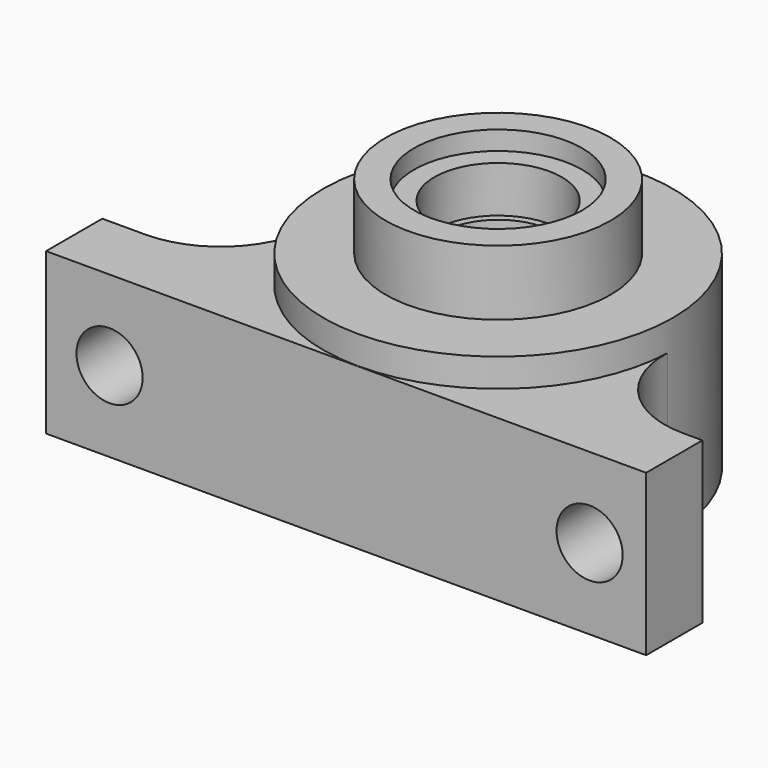
from build123d import *

# Parameters (mm, degrees)
F1_DEPTH    = 17
F3_DEPTH    = 9.5
F4_DEPTH    = 2
F5_R        = 15.5
F5_R_2      = 6
F6_DEPTH    = 3
F7_R        = 11.9
F7_R_2      = 8.9
F8_DEPTH    = 6.9
F9_T1_DEPTH = 17
F10_R       = 3.5
F11_DEPTH   = 37.0302756021
F13_DEPTH   = 29.5909779782
F14_R       = 6
F15_DEPTH   = 29.5909779782
F7_R_3      = 6.75
F16_DEPTH   = 4.9


# Not quite as in the source:
# - a fillet or chamfer that OpenCascade refuses, or shapes differently, is made with other operations: its cross-section is extruded or revolved along the edge and cut away or added
# - a feature names something its author has since deleted; it is built from what else it names


with BuildPart() as f1:
    # F0 (on Top) → F1 (new body)
    with BuildSketch(Plane.XY):
        with BuildLine():
            ThreePointArc((0, -15.5), (-5.8461671777, -14.3552195849), (-10.8287759439, -11.0899779782))
            Line((-10.8287759439, -11.0899779782), (-14.8075112171, -11.0899779782))
            ThreePointArc((-14.8075112171, -11.0899779782), (-12.6472106411, -13.5017799938), (-10.0995049384, -15.5))
            Line((-10.0995049384, -15.5), (0, -15.5))
        make_face()
        with BuildLine():
            Line((14.8075112171, -11.0899779782), (10.8287759439, -11.0899779782))
            ThreePointArc((10.8287759439, -11.0899779782), (5.8461671777, -14.3552195849), (0, -15.5))
            Line((0, -15.5), (10.0995049384, -15.5))
            ThreePointArc((10.0995049384, -15.5), (12.6472106411, -13.5017799938), (14.8075112171, -11.0899779782))
        make_face()
        with BuildLine():
            ThreePointArc((-10.8287759439, -11.0899779782), (-6.0168086586, 14.2845375692), (15.5, 0))
            ThreePointArc((15.5, 0), (14.2845375692, -6.0168086586), (10.8287759439, -11.0899779782))
            Line((10.8287759439, -11.0899779782), (14.8075112171, -11.0899779782))
            ThreePointArc((14.8075112171, -11.0899779782), (17.5526202818, -5.8442725161), (18.5, 0))
            ThreePointArc((18.5, 0), (-5.8442725161, 17.5526202818), (-14.8075112171, -11.0899779782))
            Line((-14.8075112171, -11.0899779782), (-10.8287759439, -11.0899779782))
        make_face()
        with BuildLine():
            Line((30.4899009168, -15.5), (10.0995049384, -15.5))
            ThreePointArc((10.0995049384, -15.5), (0, -18.5), (-10.0995049384, -15.5))
            Line((-10.0995049384, -15.5), (-33.0100990832, -15.5))
            Line((-33.0100990832, -15.5), (-33.0100990832, -18.5292756021))
            Line((-33.0100990832, -18.5292756021), (30.4899009168, -18.5292756021))
            Line((30.4899009168, -18.5292756021), (30.4899009168, -15.5))
        make_face()
        with BuildLine():
            Line((30.4899009168, -11.0899779782), (14.8075112171, -11.0899779782))
            ThreePointArc((14.8075112171, -11.0899779782), (12.6472106411, -13.5017799938), (10.0995049384, -15.5))
            Line((10.0995049384, -15.5), (30.4899009168, -15.5))
            Line((30.4899009168, -15.5), (30.4899009168, -11.0899779782))
        make_face()
        with BuildLine():
            ThreePointArc((-10.0995049384, -15.5), (-12.6472106411, -13.5017799938), (-14.8075112171, -11.0899779782))
            Line((-14.8075112171, -11.0899779782), (-33.0100990832, -11.0899779782))
            Line((-33.0100990832, -11.0899779782), (-33.0100990832, -15.5))
            Line((-33.0100990832, -15.5), (-10.0995049384, -15.5))
        make_face()
        with BuildLine():
            Line((10.0995049384, -15.5), (0, -15.5))
            Line((0, -15.5), (-10.0995049384, -15.5))
            ThreePointArc((-10.0995049384, -15.5), (0, -18.5), (10.0995049384, -15.5))
        make_face()
    extrude(amount=F1_DEPTH)

    # F5 (on face) → F6 (join)
    with BuildSketch(Plane.XY.offset(17)):
        with BuildLine():
            ThreePointArc((14.8075112171, -11.0899779782), (17.5526202818, -5.8442725161), (18.5, 0))
            ThreePointArc((18.5, 0), (-5.8442725161, 17.5526202818), (-14.8075112171, -11.0899779782))
            ThreePointArc((-14.8075112171, -11.0899779782), (0, -18.5), (14.8075112171, -11.0899779782))
        make_face()
        Circle(F5_R, mode=Mode.SUBTRACT)
        Circle(F5_R)
        Circle(F5_R_2, mode=Mode.SUBTRACT)
    extrude(amount=F6_DEPTH)

    # F7 (on face) → F8 (join)
    with BuildSketch(Plane.XY.offset(20)):
        Circle(F7_R)
        Circle(F7_R_2, mode=Mode.SUBTRACT)
    extrude(amount=F8_DEPTH)

    # F9: fillet of radius 10 on 2 edges, made by hand

    # F9_s2 → F9_t1 (join)
    with BuildSketch(Plane.XY):
        with BuildLine():
            ThreePointArc((18.486465371, -0.7075295648), (21.2741342918, -8.0245116996), (28.4791493554, -11.0899779782))
            Line((28.4791493554, -11.0899779782), (14.8075112171, -11.0899779782))
            ThreePointArc((14.8075112171, -11.0899779782), (17.4376325236, -6.1789134946), (18.486465371, -0.7075295648))
        make_face()
        with BuildLine():
            ThreePointArc((-18.486465371, -0.7075295648), (-21.2741342918, -8.0245116996), (-28.4791493554, -11.0899779782))
            Line((-28.4791493554, -11.0899779782), (-14.8075112171, -11.0899779782))
            ThreePointArc((-14.8075112171, -11.0899779782), (-17.4376325236, -6.1789134946), (-18.486465371, -0.7075295648))
        make_face()
    extrude(amount=F9_T1_DEPTH)

    # F10 (on face) → F11 (cut, through all)
    with BuildSketch(Plane.XZ.offset(18.5292756021)):
        with Locations((-26.2949950993, 8.5148541257)):
            Circle(F10_R)
        with Locations((24.5050049007, 8.5148541257)):
            Circle(F10_R)
    extrude(amount=-F11_DEPTH, mode=Mode.SUBTRACT)

    # F12 (on face) → F13 (cut, through all)
    with BuildSketch(Plane(origin=(0, -11.0899779782, 0), x_dir=(-1, 0, 0), z_dir=(0, 1, 0))):
        with BuildLine():
            Line((28.4791493554, 11.2497161305), (28.4791493554, 14.1031875253))
            ThreePointArc((28.4791493554, 14.1031875253), (20.2949950993, 8.5148541257), (28.4791493554, 2.926520726))
            Line((28.4791493554, 2.926520726), (28.4791493554, 5.7799921208))
            ThreePointArc((28.4791493554, 5.7799921208), (29.7949950993, 8.5148541257), (28.4791493554, 11.2497161305))
        make_face()
        with BuildLine():
            ThreePointArc((28.4791493554, 2.926520726), (31.2500392735, 5.1314331894), (32.2949950993, 8.5148541257))
            ThreePointArc((32.2949950993, 8.5148541257), (31.2500392735, 11.8982750619), (28.4791493554, 14.1031875253))
            Line((28.4791493554, 14.1031875253), (28.4791493554, 11.2497161305))
            ThreePointArc((28.4791493554, 11.2497161305), (29.7949950993, 8.5148541257), (28.4791493554, 5.7799921208))
            Line((28.4791493554, 5.7799921208), (28.4791493554, 2.926520726))
        make_face()
    extrude(amount=F13_DEPTH, mode=Mode.SUBTRACT)

    # F14 (on face) → F15 (cut, through all)
    with BuildSketch(Plane(origin=(0, -11.0899779782, 0), x_dir=(-1, 0, 0), z_dir=(0, 1, 0))):
        with Locations((-24.5050049007, 8.5148541257)):
            Circle(F14_R)
    extrude(amount=F15_DEPTH, mode=Mode.SUBTRACT)

    # F7 (on face) → F16 (join)
    with BuildSketch(Plane.XY.offset(20)):
        Circle(F7_R_2)
        Circle(F7_R_3, mode=Mode.SUBTRACT)
    extrude(amount=F16_DEPTH)


with BuildPart() as f3:
    # F2 (on face) → F3 (new body)
    with BuildSketch(Plane.XY.offset(17)):
        with BuildLine():
            Line((10.7419644717, 11.1740860605), (7.5760127927, 8.651822361))
            ThreePointArc((7.5760127927, 8.651822361), (10.473159674, 4.7500448884), (11.5, 0))
            ThreePointArc((11.5, 0), (8.5603531215, -7.6792157435), (1.2442861853, -11.4324866888))
            Line((1.2442861853, -11.4324866888), (2.0058842699, -15.3696593422))
            ThreePointArc((2.0058842699, -15.3696593422), (11.6477724519, -10.2264068425), (15.5, 0))
            ThreePointArc((15.5, 0), (14.2609685735, 6.0724604029), (10.7419644717, 11.1740860605))
        make_face()
        with BuildLine():
            Line((0.8345908665, 15.4775145965), (1.1546689089, 11.4418853215))
            ThreePointArc((1.1546689089, 11.4418853215), (4.5828281197, 10.5474018803), (7.5760127927, 8.651822361))
            Line((7.5760127927, 8.651822361), (10.7419644717, 11.1740860605))
            ThreePointArc((10.7419644717, 11.1740860605), (6.1752759182, 14.2167495348), (0.8345908665, 15.4775145965))
        make_face()
        with BuildLine():
            ThreePointArc((-8.0347933894, 8.2275205979), (-3.7969808217, 10.855088053), (1.1546689089, 11.4418853215))
            Line((1.1546689089, 11.4418853215), (0.8345908665, 15.4775145965))
            ThreePointArc((0.8345908665, 15.4775145965), (-5.2813630167, 14.5724810752), (-10.5570475908, 11.3489535274))
            Line((-10.5570475908, 11.3489535274), (-8.0347933894, 8.2275205979))
        make_face()
        with BuildLine():
            ThreePointArc((1.2442861853, -11.4324866888), (-10.3998422416, -4.9084907405), (-8.0347933894, 8.2275205979))
            Line((-8.0347933894, 8.2275205979), (-10.5570475908, 11.3489535274))
            ThreePointArc((-10.5570475908, 11.3489535274), (-14.0268195595, -6.5953266065), (2.0058842699, -15.3696593422))
            Line((2.0058842699, -15.3696593422), (1.2442861853, -11.4324866888))
        make_face()
    extrude(amount=-F3_DEPTH)

    # F2 (on face) → F4 (join)
    with BuildSketch(Plane.XY.offset(17)):
        with BuildLine():
            Line((-3.9074059307, 3.119644033), (-8.0347933894, 8.2275205979))
            ThreePointArc((-8.0347933894, 8.2275205979), (-10.3998422416, -4.9084907405), (1.2442861853, -11.4324866888))
            Line((1.2442861853, -11.4324866888), (0, -5))
            ThreePointArc((0, -5), (-4.5054533715, -2.1681535733), (-3.9074059307, 3.119644033))
        make_face()
        with BuildLine():
            Line((1.1546689089, 11.4418853215), (1.3564967681, 8.8971858763))
            ThreePointArc((1.3564967681, 8.8971858763), (3.5875748475, 8.2540478987), (5.5798650145, 7.0615229533))
            Line((5.5798650145, 7.0615229533), (7.5760127927, 8.651822361))
            ThreePointArc((7.5760127927, 8.651822361), (4.5828281197, 10.5474018803), (1.1546689089, 11.4418853215))
        make_face()
    extrude(amount=-F4_DEPTH)


solid = Compound([f1.part, f3.part])
